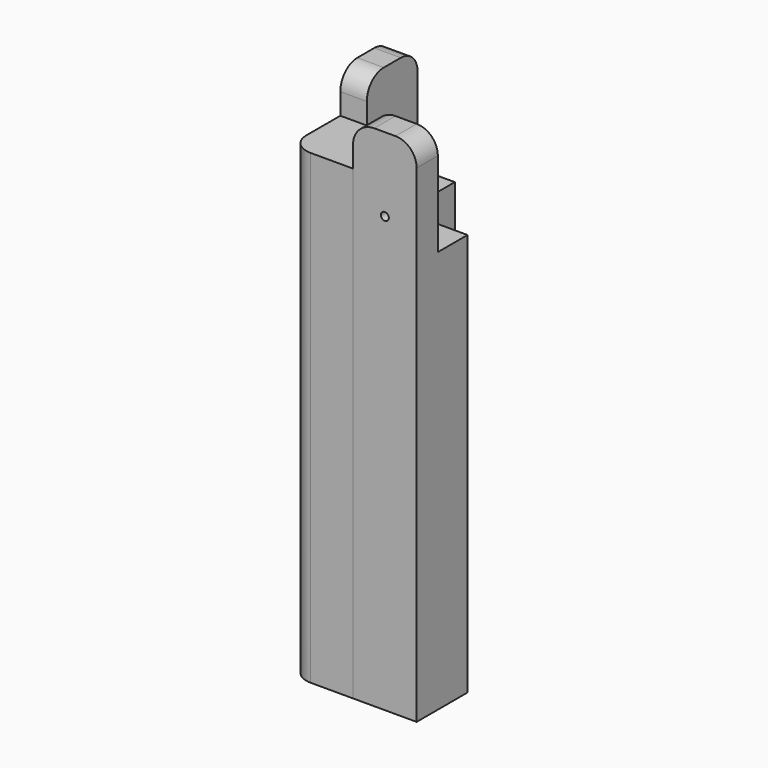
from build123d import *

# Parameters (mm, degrees)
F0_W      = 76.2
F0_H      = 76.2
F1_DEPTH  = 558.8
F4_DEPTH  = 50.8
F5_DEPTH  = 50.8
F6_W      = 44.45
F6_H      = 76.2
F7_DEPTH  = 127
F8_W      = 76.2
F8_H      = 44.45
F9_DEPTH  = 127
F10_R     = 25.4
F10_2_R   = 25.4
F10_3_R   = 25.4
F11_R     = 4.7625
F12_DEPTH = 31.751
F13_R     = 4.7625
F14_DEPTH = 31.751


with BuildPart() as f1:
    # F0 (on Top) → F1 (new body)
    with BuildSketch(Plane.XY):
        with Locations((38.1, 38.1)):
            Rectangle(F0_W, F0_H)
    extrude(amount=F1_DEPTH)


with BuildPart() as f2_1:
    # F2: copy of F1
    add(f1.part.moved(Location((76.2, 0, 0))))

    # F5 (add): a face of the model
    f5_faces = [f2_1.faces().sort_by_distance(p)[0] for p in [
        (114.3, 38.1, 558.8),
    ]]
    extrude(f5_faces, amount=F5_DEPTH)

    # F8 (on face) → F9 (cut)
    with BuildSketch(Plane.XY.offset(609.6)):
        with Locations((114.3, 53.975)):
            Rectangle(F8_W, F8_H)
    extrude(amount=-F9_DEPTH, mode=Mode.SUBTRACT)

    # F10#2
    f10_2_edges = [f2_1.edges().sort_by_distance(p)[0] for p in [
        (76.2, 15.875, 609.6),
        (152.4, 15.875, 609.6),
    ]]
    fillet(f10_2_edges, radius=F10_2_R)

    # F13 (on face) → F14 (cut, through all)
    with BuildSketch(Plane(origin=(0, 31.75, 0), x_dir=(-1, 0, 0), z_dir=(0, 1, 0))):
        with Locations((-114.3, 520.7)):
            Circle(F13_R)
    extrude(amount=-F14_DEPTH, mode=Mode.SUBTRACT)


with BuildPart() as f3_1:
    # F3: copy of F1
    add(f1.part.moved(Location((0, 76.2, 0))))

    # F4 (add): a face of the model
    f4_faces = [f3_1.faces().sort_by_distance(p)[0] for p in [
        (38.1, 114.3, 558.8),
    ]]
    extrude(f4_faces, amount=F4_DEPTH)

    # F6 (on face) → F7 (cut)
    with BuildSketch(Plane.XY.offset(609.6)):
        with Locations((53.975, 114.3)):
            Rectangle(F6_W, F6_H)
    extrude(amount=-F7_DEPTH, mode=Mode.SUBTRACT)

    # F10#3
    f10_3_edges = [f3_1.edges().sort_by_distance(p)[0] for p in [
        (15.875, 76.2, 609.6),
        (15.875, 152.4, 609.6),
    ]]
    fillet(f10_3_edges, radius=F10_3_R)

    # F11 (on face) → F12 (cut, through all)
    with BuildSketch(Plane.YZ.offset(31.75)):
        with Locations((114.3, 520.7)):
            Circle(F11_R)
    extrude(amount=-F12_DEPTH, mode=Mode.SUBTRACT)


with BuildPart() as f1_1:
    add(f1.part)

    # F10
    f10_edges = [f1_1.edges().sort_by_distance(p)[0] for p in [
        (0, 0, 279.4),
    ]]
    fillet(f10_edges, radius=F10_R)


solid = Compound([f2_1.part, f3_1.part, f1_1.part])
